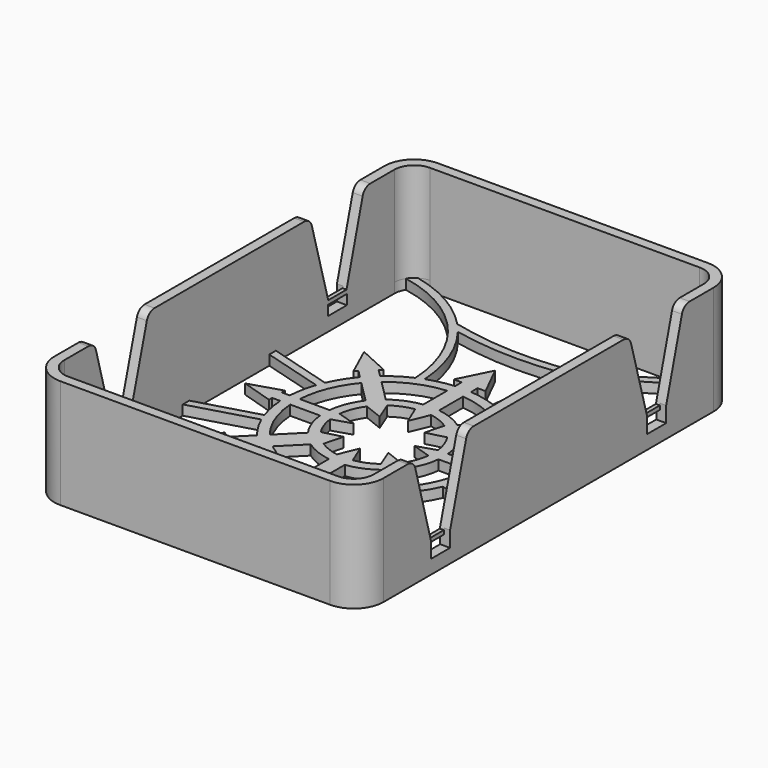
from build123d import *

# Parameters (mm, degrees)
F1_DEPTH  = 2.5
F3_DEPTH  = 25
F4_W      = 6
F4_H      = 2.5
F5_DEPTH  = 100
F6_R      = 2.5
F7_W      = 6
F7_H      = 1.6
F8_DEPTH  = 1.5
F9_W      = 6
F9_H      = 1.6
F10_DEPTH = 1.5
F11_W     = 6
F11_H     = 1.6
F12_DEPTH = 1.5


# Not quite as in the source:
# - a feature names something its author has since deleted; it is built from what else it names


with BuildPart() as f1:
    # F0 (on Top) → F1 (new body)
    with BuildSketch(Plane.XY):
        with BuildLine():
            Line((34, 59.5), (-34, 59.5))
            ThreePointArc((-34, 59.5), (-39.3033008589, 57.3033008589), (-41.5, 52))
            Line((-41.5, 52), (-41.5, -52))
            ThreePointArc((-41.5, -52), (-39.3033008589, -57.3033008589), (-34, -59.5))
            Line((-34, -59.5), (34, -59.5))
            ThreePointArc((34, -59.5), (39.3033008589, -57.3033008589), (41.5, -52))
            Line((41.5, -52), (41.5, 52))
            ThreePointArc((41.5, 52), (39.3033008589, 57.3033008589), (34, 59.5))
        make_face()
        with BuildLine():
            ThreePointArc((-10.3121841573, -22.7740830311), (-18.7546988225, -43.5494396608), (-38.2378445577, -54.6534267475))
            ThreePointArc((-38.2378445577, -54.6534267475), (-38.8056853199, -53.380358144), (-39, -52))
            Line((-39, -52), (-39, -14.6753967433))
            Line((-39, -14.6753967433), (-22.8991444466, -10.0314098518))
            ThreePointArc((-22.8991444466, -10.0314098518), (-21.3253943679, -13.0471282301), (-19.3568260523, -15.8212921464))
            Line((-19.3568260523, -15.8212921464), (-23.6880771697, -20.1525432638))
            Line((-23.6880771697, -20.1525432638), (-25.1022907321, -18.7383297014))
            Line((-25.1022907321, -18.7383297014), (-28.2842712475, -28.2842712475))
            Line((-28.2842712475, -28.2842712475), (-18.7383297014, -25.1022907321))
            Line((-18.7383297014, -25.1022907321), (-20.1525432638, -23.6880771697))
            Line((-20.1525432638, -23.6880771697), (-15.8212921464, -19.3568260523))
            ThreePointArc((-15.8212921464, -19.3568260523), (-13.1779762196, -21.2447862488), (-10.3121841573, -22.7740830311))
        make_face(mode=Mode.SUBTRACT)
        with BuildLine():
            Line((-14.0436213479, -17.5791552538), (-8.6904833787, -12.2260172846))
            ThreePointArc((-8.6904833787, -12.2260172846), (-5.5058220684, -13.9529897639), (-2, -14.8660687473))
            Line((-2, -14.8660687473), (-2, -22.410934831))
            ThreePointArc((-2, -22.410934831), (-8.3777067243, -20.8821462029), (-14.0436213479, -17.5791552538))
        make_face(mode=Mode.SUBTRACT)
        with BuildLine():
            ThreePointArc((-14.9248115566, -1.5), (-14.0434197935, -5.2708975046), (-12.2260172846, -8.6904833787))
            Line((-12.2260172846, -8.6904833787), (-17.5791552538, -14.0436213479))
            ThreePointArc((-17.5791552538, -14.0436213479), (-20.9742177998, -8.1444574825), (-22.4499443206, -1.5))
            Line((-22.4499443206, -1.5), (-14.9248115566, -1.5))
        make_face(mode=Mode.SUBTRACT)
        with BuildLine():
            Line((34, -57), (-34, -57))
            ThreePointArc((-34, -57), (-35.2900266724, -56.8307174606), (-36.4927017485, -56.3343324738))
            ThreePointArc((-36.4927017485, -56.3343324738), (-26.5730446815, -52.4657558123), (-18.2188270759, -45.8648066449))
            ThreePointArc((-18.2188270759, -45.8648066449), (0.0645372678, -43.6548366659), (18.3480120928, -45.8638924263))
            ThreePointArc((18.3480120928, -45.8638924263), (26.6444809001, -52.4472652568), (36.4976568405, -56.3314789977))
            ThreePointArc((36.4976568405, -56.3314789977), (35.2927886548, -56.8299790366), (34, -57))
        make_face(mode=Mode.SUBTRACT)
        with BuildLine():
            Line((-2, -24.9198715888), (-2, -27))
            Line((-2, -27), (-4, -27))
            Line((-4, -27), (0, -35))
            Line((0, -35), (4, -27))
            Line((4, -27), (2, -27))
            Line((2, -27), (2, -24.9198715888))
            ThreePointArc((2, -24.9198715888), (5.3990366559, -24.4100471771), (8.6960239938, -23.4388388513))
            ThreePointArc((8.6960239938, -23.4388388513), (10.9380944649, -33.944555482), (16.1801351306, -43.3210138528))
            ThreePointArc((16.1801351306, -43.3210138528), (0.0679407898, -41.6548366559), (-16.0443163621, -43.3204063469))
            ThreePointArc((-16.0443163621, -43.3204063469), (-10.8003212907, -33.972941987), (-8.5406637385, -23.4958945968))
            ThreePointArc((-8.5406637385, -23.4958945968), (-5.3182069939, -24.4277848846), (-2, -24.9198715888))
        make_face(mode=Mode.SUBTRACT)
        with BuildLine():
            ThreePointArc((39, -52), (38.8053271602, -53.38160446), (38.2364676465, -54.6556245744))
            ThreePointArc((38.2364676465, -54.6556245744), (18.8416922801, -43.4650136984), (10.5463986385, -22.666571769))
            ThreePointArc((10.5463986385, -22.666571769), (13.4992605836, -21.042099793), (16.2067966243, -19.0352237491))
            Line((16.2067966243, -19.0352237491), (18.0566773959, -20.8851045206))
            Line((18.0566773959, -20.8851045206), (17.3495706147, -21.5922113018))
            Line((17.3495706147, -21.5922113018), (25.1277452077, -25.1277452077))
            Line((25.1277452077, -25.1277452077), (21.5922113018, -17.3495706147))
            Line((21.5922113018, -17.3495706147), (20.8851045206, -18.0566773959))
            Line((20.8851045206, -18.0566773959), (19.0352237491, -16.2067966243))
            ThreePointArc((19.0352237491, -16.2067966243), (21.1933163861, -13.2605935221), (22.8991444466, -10.0314098518))
            Line((22.8991444466, -10.0314098518), (39, -14.6753967433))
            Line((39, -14.6753967433), (39, -52))
        make_face(mode=Mode.SUBTRACT)
        with BuildLine():
            ThreePointArc((2, -14.8660687473), (5.7402514855, -13.8581929877), (9.0976844584, -11.9261115832))
            Line((9.0976844584, -11.9261115832), (14.4327104294, -17.2611375541))
            ThreePointArc((14.4327104294, -17.2611375541), (8.6103772282, -20.7872894815), (2, -22.410934831))
            Line((2, -22.410934831), (2, -14.8660687473))
        make_face(mode=Mode.SUBTRACT)
        with BuildLine():
            ThreePointArc((22.4499443206, -1.5), (20.8819600536, -8.3781707026), (17.2611375541, -14.4327104294))
            Line((17.2611375541, -14.4327104294), (11.9261115832, -9.0976844584))
            ThreePointArc((11.9261115832, -9.0976844584), (13.9525703957, -5.506884723), (14.9248115566, -1.5))
            Line((14.9248115566, -1.5), (22.4499443206, -1.5))
        make_face(mode=Mode.SUBTRACT)
        with BuildLine():
            Line((-24.9549594269, 1.5), (-27, 1.5))
            Line((-27, 1.5), (-27, 2.5))
            Line((-27, 2.5), (-35, 0))
            Line((-35, 0), (-27, -2.5))
            Line((-27, -2.5), (-27, -1.5))
            Line((-27, -1.5), (-24.9549594269, -1.5))
            ThreePointArc((-24.9549594269, -1.5), (-24.5199625183, -4.8755961791), (-23.6305078429, -8.160827108))
            Line((-23.6305078429, -8.160827108), (-39, -12.5938660772))
            Line((-39, -12.5938660772), (-39, 12.5938660772))
            Line((-39, 12.5938660772), (-23.6305078429, 8.160827108))
            ThreePointArc((-23.6305078429, 8.160827108), (-24.5199625183, 4.8755961791), (-24.9549594269, 1.5))
        make_face(mode=Mode.SUBTRACT)
        with BuildLine():
            Line((-17.2611375541, 14.4327104294), (-11.9261115832, 9.0976844584))
            ThreePointArc((-11.9261115832, 9.0976844584), (-13.9525703957, 5.506884723), (-14.9248115566, 1.5))
            Line((-14.9248115566, 1.5), (-22.4499443206, 1.5))
            ThreePointArc((-22.4499443206, 1.5), (-20.8819600536, 8.3781707026), (-17.2611375541, 14.4327104294))
        make_face(mode=Mode.SUBTRACT)
        with BuildLine():
            ThreePointArc((-2, 14.8660687473), (-5.7402514855, 13.8581929877), (-9.0976844584, 11.9261115832))
            Line((-9.0976844584, 11.9261115832), (-14.4327104294, 17.2611375541))
            ThreePointArc((-14.4327104294, 17.2611375541), (-8.6103772282, 20.7872894815), (-2, 22.410934831))
            Line((-2, 22.410934831), (-2, 14.8660687473))
        make_face(mode=Mode.SUBTRACT)
        with BuildLine():
            ThreePointArc((-39, 52), (-38.8056853199, 53.380358144), (-38.2378445577, 54.6534267475))
            ThreePointArc((-38.2378445577, 54.6534267475), (-18.7546988225, 43.5494396608), (-10.3121841573, 22.7740830311))
            ThreePointArc((-10.3121841573, 22.7740830311), (-13.3906255495, 21.1113985182), (-16.2067966243, 19.0352237491))
            Line((-16.2067966243, 19.0352237491), (-18.0566773959, 20.8851045206))
            Line((-18.0566773959, 20.8851045206), (-17.3495706147, 21.5922113018))
            Line((-17.3495706147, 21.5922113018), (-25.1277452077, 25.1277452077))
            Line((-25.1277452077, 25.1277452077), (-21.5922113018, 17.3495706147))
            Line((-21.5922113018, 17.3495706147), (-20.8851045206, 18.0566773959))
            Line((-20.8851045206, 18.0566773959), (-19.0352237491, 16.2067966243))
            ThreePointArc((-19.0352237491, 16.2067966243), (-21.1933163861, 13.2605935221), (-22.8991444466, 10.0314098518))
            Line((-22.8991444466, 10.0314098518), (-39, 14.6753967433))
            Line((-39, 14.6753967433), (-39, 52))
        make_face(mode=Mode.SUBTRACT)
        with BuildLine():
            ThreePointArc((-2, -12.3389626793), (-4.5477473735, -11.6433669455), (-6.8924870849, -10.4280209908))
            Line((-6.8924870849, -10.4280209908), (-5.6556002237, -5.6556002237))
            Line((-5.6556002237, -5.6556002237), (-10.4280209908, -6.8924870849))
            ThreePointArc((-10.4280209908, -6.8924870849), (-11.7328514574, -4.3116350354), (-12.409673646, -1.5))
            Line((-12.409673646, -1.5), (-7.6522814424, 0))
            Line((-7.6522814424, 0), (-12.409673646, 1.5))
            ThreePointArc((-12.409673646, 1.5), (-11.642760861, 4.5492987959), (-10.1391777457, 7.3107506209))
            Line((-10.1391777457, 7.3107506209), (-5.4715881124, 5.4715881124))
            Line((-5.4715881124, 5.4715881124), (-7.3107506209, 10.1391777457))
            ThreePointArc((-7.3107506209, 10.1391777457), (-4.7835429046, 11.5484941564), (-2, 12.3389626793))
            Line((-2, 12.3389626793), (0, 7.5105355545))
            Line((0, 7.5105355545), (2, 12.3389626793))
            ThreePointArc((2, 12.3389626793), (4.5477473735, 11.6433669455), (6.8924870849, 10.4280209908))
            Line((6.8924870849, 10.4280209908), (5.6556002237, 5.6556002237))
            Line((5.6556002237, 5.6556002237), (10.4280209908, 6.8924870849))
            ThreePointArc((10.4280209908, 6.8924870849), (11.7328514574, 4.3116350354), (12.409673646, 1.5))
            Line((12.409673646, 1.5), (7.6522814424, 0))
            Line((7.6522814424, 0), (12.409673646, -1.5))
            ThreePointArc((12.409673646, -1.5), (11.642760861, -4.5492987959), (10.1391777457, -7.3107506209))
            Line((10.1391777457, -7.3107506209), (5.4715881124, -5.4715881124))
            Line((5.4715881124, -5.4715881124), (7.3107506209, -10.1391777457))
            ThreePointArc((7.3107506209, -10.1391777457), (4.7835429046, -11.5484941564), (2, -12.3389626793))
            Line((2, -12.3389626793), (0, -7.5105355545))
            Line((0, -7.5105355545), (-2, -12.3389626793))
        make_face(mode=Mode.SUBTRACT)
        with BuildLine():
            ThreePointArc((14.9248115566, 1.5), (14.0434197935, 5.2708975046), (12.2260172846, 8.6904833787))
            Line((12.2260172846, 8.6904833787), (17.5791552538, 14.0436213479))
            ThreePointArc((17.5791552538, 14.0436213479), (20.9742177998, 8.1444574825), (22.4499443206, 1.5))
            Line((22.4499443206, 1.5), (14.9248115566, 1.5))
        make_face(mode=Mode.SUBTRACT)
        with BuildLine():
            ThreePointArc((8.6904833787, 12.2260172846), (5.5058220684, 13.9529897639), (2, 14.8660687473))
            Line((2, 14.8660687473), (2, 22.410934831))
            ThreePointArc((2, 22.410934831), (8.3777067243, 20.8821462029), (14.0436213479, 17.5791552538))
            Line((14.0436213479, 17.5791552538), (8.6904833787, 12.2260172846))
        make_face(mode=Mode.SUBTRACT)
        with BuildLine():
            Line((27, 2.5), (27, 1.5))
            Line((27, 1.5), (24.9549594269, 1.5))
            ThreePointArc((24.9549594269, 1.5), (24.5199625183, 4.8755961791), (23.6305078429, 8.160827108))
            Line((23.6305078429, 8.160827108), (39, 12.5938660772))
            Line((39, 12.5938660772), (39, -12.5938660772))
            Line((39, -12.5938660772), (23.6305078429, -8.160827108))
            ThreePointArc((23.6305078429, -8.160827108), (24.5199625183, -4.8755961791), (24.9549594269, -1.5))
            Line((24.9549594269, -1.5), (27, -1.5))
            Line((27, -1.5), (27, -2.5))
            Line((27, -2.5), (35, 0))
            Line((35, 0), (27, 2.5))
        make_face(mode=Mode.SUBTRACT)
        with BuildLine():
            Line((4, 27), (0, 35))
            Line((0, 35), (-4, 27))
            Line((-4, 27), (-2, 27))
            Line((-2, 27), (-2, 24.9198715888))
            ThreePointArc((-2, 24.9198715888), (-5.3182069939, 24.4277848846), (-8.5406637385, 23.4958945968))
            ThreePointArc((-8.5406637385, 23.4958945968), (-10.8003212907, 33.972941987), (-16.0443163621, 43.3204063469))
            ThreePointArc((-16.0443163621, 43.3204063469), (0.0679407898, 41.6548366559), (16.1801351306, 43.3210138528))
            ThreePointArc((16.1801351306, 43.3210138528), (10.9380944649, 33.944555482), (8.6960239938, 23.4388388513))
            ThreePointArc((8.6960239938, 23.4388388513), (5.3990366559, 24.4100471771), (2, 24.9198715888))
            Line((2, 24.9198715888), (2, 27))
            Line((2, 27), (4, 27))
        make_face(mode=Mode.SUBTRACT)
        with BuildLine():
            ThreePointArc((-36.4927017485, 56.3343324738), (-35.2900266724, 56.8307174606), (-34, 57))
            Line((-34, 57), (34, 57))
            ThreePointArc((34, 57), (35.2927886548, 56.8299790366), (36.4976568405, 56.3314789977))
            ThreePointArc((36.4976568405, 56.3314789977), (26.6444809001, 52.4472652568), (18.3480120928, 45.8638924263))
            ThreePointArc((18.3480120928, 45.8638924263), (0.0645372678, 43.6548366659), (-18.2188270759, 45.8648066449))
            ThreePointArc((-18.2188270759, 45.8648066449), (-26.5730446815, 52.4657558123), (-36.4927017485, 56.3343324738))
        make_face(mode=Mode.SUBTRACT)
        with BuildLine():
            ThreePointArc((10.5463986385, 22.666571769), (18.8416922801, 43.4650136984), (38.2364676465, 54.6556245744))
            ThreePointArc((38.2364676465, 54.6556245744), (38.8053271602, 53.38160446), (39, 52))
            Line((39, 52), (39, 14.6753967433))
            Line((39, 14.6753967433), (22.8991444466, 10.0314098518))
            ThreePointArc((22.8991444466, 10.0314098518), (21.3253943679, 13.0471282301), (19.3568260523, 15.8212921464))
            Line((19.3568260523, 15.8212921464), (23.6880771697, 20.1525432638))
            Line((23.6880771697, 20.1525432638), (25.1022907321, 18.7383297014))
            Line((25.1022907321, 18.7383297014), (28.2842712475, 28.2842712475))
            Line((28.2842712475, 28.2842712475), (18.7383297014, 25.1022907321))
            Line((18.7383297014, 25.1022907321), (20.1525432638, 23.6880771697))
            Line((20.1525432638, 23.6880771697), (15.8212921464, 19.3568260523))
            ThreePointArc((15.8212921464, 19.3568260523), (13.2873015887, 21.1765817943), (10.5463986385, 22.666571769))
        make_face(mode=Mode.SUBTRACT)
    extrude(amount=F1_DEPTH)

    # F2 (on face) → F3 (join)
    with BuildSketch(Plane.XY.offset(2.5)):
        with BuildLine():
            Line((34, 59.5), (-34, 59.5))
            ThreePointArc((-34, 59.5), (-39.3033008589, 57.3033008589), (-41.5, 52))
            Line((-41.5, 52), (-41.5, -52))
            ThreePointArc((-41.5, -52), (-39.3033008589, -57.3033008589), (-34, -59.5))
            Line((-34, -59.5), (34, -59.5))
            ThreePointArc((34, -59.5), (39.3033008589, -57.3033008589), (41.5, -52))
            Line((41.5, -52), (41.5, 52))
            ThreePointArc((41.5, 52), (39.3033008589, 57.3033008589), (34, 59.5))
        make_face()
        with BuildLine():
            ThreePointArc((-39, 52), (-37.5355339059, 55.5355339059), (-34, 57))
            Line((-34, 57), (34, 57))
            ThreePointArc((34, 57), (37.5355339059, 55.5355339059), (39, 52))
            Line((39, 52), (39, -52))
            ThreePointArc((39, -52), (37.5355339059, -55.5355339059), (34, -57))
            Line((34, -57), (-34, -57))
            ThreePointArc((-34, -57), (-37.5355339059, -55.5355339059), (-39, -52))
            Line((-39, -52), (-39, 52))
        make_face(mode=Mode.SUBTRACT)
    extrude(amount=F3_DEPTH)

    # F4 (on face) → F5 (cut)
    with BuildSketch(Plane.YZ.offset(41.5)):
        Polygon((-36.9336101614, 7), (-31.1714837525, 7), (-25.4810947511, 27.5), (-42.5182211601, 27.5), align=None)
        with Locations((-34.0515990257, 4.75)):
            Rectangle(F4_W, F4_H)
        Polygon((36.9336101614, 7), (42.5182211601, 27.5), (25.4810947511, 27.5), (31.1714837525, 7), align=None)
        with Locations((34.0515990257, 4.75)):
            Rectangle(F4_W, F4_H)
    extrude(amount=-F5_DEPTH, mode=Mode.SUBTRACT)

    # F6
    f6_edges = [f1.edges().sort_by_distance(p)[0] for p in [
        (40.25, 42.518221, 27.5),
        (-40.25, 42.518221, 27.5),
        (40.25, 25.481095, 27.5),
        (40.25, -25.481095, 27.5),
        (40.25, -42.518221, 27.5),
        (-40.25, -42.518221, 27.5),
        (-40.25, 25.481095, 27.5),
        (-40.25, -25.481095, 27.5),
    ]]
    fillet(f6_edges, radius=F6_R)

    # F7 (on face) → F8 (cut)
    with BuildSketch(Plane.YZ.offset(41.5)):
        with Locations((-34.0515990257, 6.8)):
            Rectangle(F7_W, F7_H)
    extrude(amount=-F8_DEPTH, mode=Mode.SUBTRACT)

    # F9 (on face) → F10 (cut)
    with BuildSketch(Plane.YZ.offset(41.5)):
        with Locations((34.0515990257, 6.8)):
            Rectangle(F9_W, F9_H)
    extrude(amount=-F10_DEPTH, mode=Mode.SUBTRACT)

    # F11 (on face) → F12 (cut)
    with BuildSketch(Plane(origin=(-41.5, 0, 0), x_dir=(0, -1, 0), z_dir=(-1, 0, 0))):
        with Locations((-34.0515990257, 6.8)):
            Rectangle(F11_W, F11_H)
        with Locations((34.0515990257, 6.8)):
            Rectangle(F11_W, F11_H)
    extrude(amount=-F12_DEPTH, mode=Mode.SUBTRACT)


solid = f1.part
